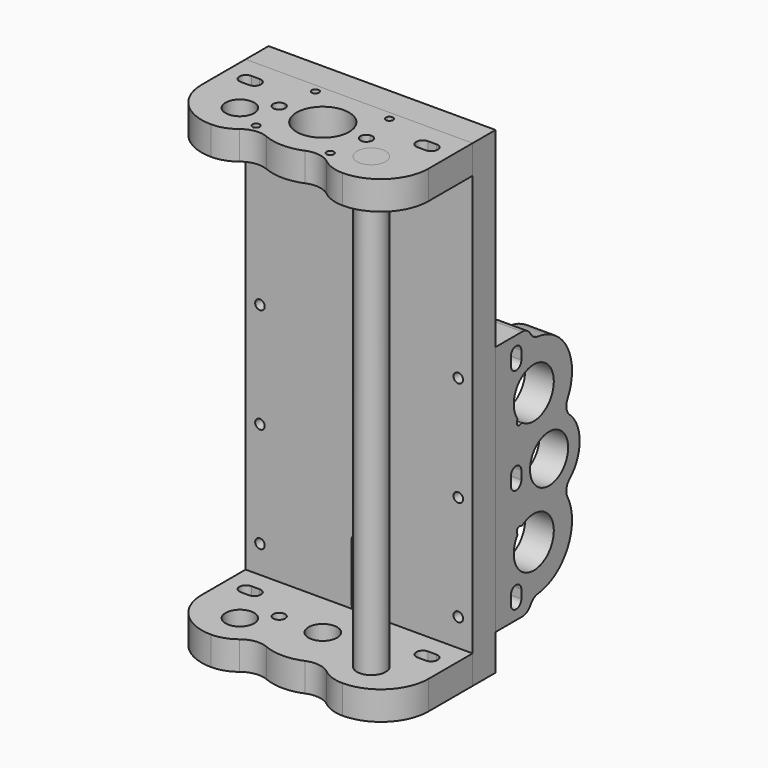
from build123d import *

# Parameters (mm, degrees)
F1_DEPTH       = 12
F2_R           = 11
F2_R_2         = 5.975
F3_DEPTH       = 12
F4_R           = 10
F5_R           = 6
F6_DEPTH       = 188
F7_R           = 9.975
F8_DEPTH       = 12
F9_R           = 2.5
F9_R_2         = 6
F9_R_3         = 5.9749995874
F10_DEPTH      = 12
F11_R          = 2
F12_DEPTH      = 25
F12_DEPTH_BACK = 10
F13_R          = 1.5
F14_DEPTH      = 25
F15_R          = 5
F16_R          = 5


# Not quite as in the source:
# - ends of sketch curves that miss each other by under 0.0002 mm in the source are joined


with BuildPart() as f1:
    # F0 (on Front) → F1 (new body)
    with BuildSketch(Plane.XZ):
        Polygon((-47.5, 1.6334e-06), (47.5, -1.6334e-06), (47.5, 200.0000016334), (-47.5, 200.0000016334), align=None)
        with BuildLine():
            ThreePointArc((3.25, 14), (0, 10.75), (-3.25, 14))
            Line((-3.25, 14), (-3.25, 37))
            ThreePointArc((-3.25, 37), (0, 40.25), (3.25, 37))
            Line((3.25, 37), (3.25, 14))
        make_face(mode=Mode.SUBTRACT)
        with BuildLine():
            ThreePointArc((-3.25, 186.0000016334), (0, 189.2500016334), (3.25, 186.0000016334))
            Line((3.25, 186.0000016334), (3.25, 163.0000016334))
            ThreePointArc((3.25, 163.0000016334), (0, 159.7500016334), (-3.25, 163.0000016334))
            Line((-3.25, 163.0000016334), (-3.25, 186.0000016334))
        make_face(mode=Mode.SUBTRACT)
    extrude(amount=-F1_DEPTH)


with BuildPart() as f3:
    # F2 (on face) → F3 (new body)
    with BuildSketch(Plane.XY.offset(200.0000016334)):
        with BuildLine():
            Line((-8.94427191, 0), (-47.5, 0))
            Line((-47.5, 0), (-47.5, -23))
            ThreePointArc((-47.5, -23), (-41.6421356237, -37.1421356237), (-27.5, -43))
            ThreePointArc((-27.5, -43), (-42.0677346215, -24.4249324484), (-20.5559152874, -14.7041477331))
            ThreePointArc((-20.5559152874, -14.7041477331), (-16.4808449816, -5.9853256402), (-8.94427191, 0))
        make_face()
        with BuildLine():
            ThreePointArc((-38.75, -13.5), (-41.5, -10.75), (-38.75, -8))
            Line((-38.75, -8), (-35.25, -8))
            ThreePointArc((-35.25, -8), (-32.5, -10.75), (-35.25, -13.5))
            Line((-35.25, -13.5), (-38.75, -13.5))
        make_face(mode=Mode.SUBTRACT)
        with BuildLine():
            Line((8.94427191, 0), (-8.94427191, 0))
            ThreePointArc((-8.94427191, 0), (-16.4808449816, -5.9853256402), (-20.5559152874, -14.7041477331))
            ThreePointArc((-20.5559152874, -14.7041477331), (-19.1407664776, -15.5451529548), (-17.8262976116, -16.5361663437))
            ThreePointArc((-17.8262976116, -16.5361663437), (-16.4581851727, -17.2566126005), (-15.7754847524, -18.6439462267))
            ThreePointArc((-15.7754847524, -18.6439462267), (-13.3425332649, -23.0435763253), (-12.5, -28))
            ThreePointArc((-12.5, -28), (-12.8897484194, -31.397138318), (-14.0387398336, -34.6177393974))
            ThreePointArc((-14.0387398336, -34.6177393974), (0, -40), (14.0387398336, -34.6177393974))
            ThreePointArc((14.0387398336, -34.6177393974), (12.587879498, -26.3786850603), (15.7754847524, -18.6439462267))
            ThreePointArc((15.7754847524, -18.6439462267), (16.4581851727, -17.2566126005), (17.8262976116, -16.5361663437))
            ThreePointArc((17.8262976116, -16.5361663437), (19.1407664776, -15.5451529548), (20.5559152874, -14.7041477331))
            ThreePointArc((20.5559152874, -14.7041477331), (16.4808449816, -5.9853256402), (8.94427191, 0))
        make_face()
        with Locations((0, -19)):
            Circle(F2_R, mode=Mode.SUBTRACT)
        with BuildLine():
            Line((47.5, 0), (8.94427191, 0))
            ThreePointArc((8.94427191, 0), (16.4808449816, -5.9853256402), (20.5559152874, -14.7041477331))
            ThreePointArc((20.5559152874, -14.7041477331), (35.2729894285, -15.1711015537), (42.5, -28))
            ThreePointArc((42.5, -28), (38.1066017178, -38.6066017178), (27.5, -43))
            ThreePointArc((27.5, -43), (41.6421356237, -37.1421356237), (47.5, -23))
            Line((47.5, -23), (47.5, 0))
        make_face()
        with BuildLine():
            Line((38.75, -13.5), (35.25, -13.5))
            ThreePointArc((35.25, -13.5), (32.5, -10.75), (35.25, -8))
            Line((35.25, -8), (38.75, -8))
            ThreePointArc((38.75, -8), (41.5, -10.75), (38.75, -13.5))
        make_face(mode=Mode.SUBTRACT)
        with BuildLine():
            ThreePointArc((-17.8262976116, -16.5361663437), (-19.1407664776, -15.5451529548), (-20.5559152874, -14.7041477331))
            ThreePointArc((-20.5559152874, -14.7041477331), (-19.9583397099, -25.5318202687), (-14.0387398336, -34.6177393974))
            ThreePointArc((-14.0387398336, -34.6177393974), (-12.8897484194, -31.397138318), (-12.5, -28))
            ThreePointArc((-12.5, -28), (-13.3425332649, -23.0435763253), (-15.7754847524, -18.6439462267))
            ThreePointArc((-15.7754847524, -18.6439462267), (-15.7563793273, -18.8215176745), (-15.75, -19))
            ThreePointArc((-15.75, -19), (-20.1617081329, -20.6110158331), (-17.8262976116, -16.5361663437))
        make_face()
        with BuildLine():
            ThreePointArc((-14.0387398336, -34.6177393974), (-19.9583397099, -25.5318202687), (-20.5559152874, -14.7041477331))
            ThreePointArc((-20.5559152874, -14.7041477331), (-42.0677346215, -24.4249324484), (-27.5, -43))
            ThreePointArc((-27.5, -43), (-19.5711315738, -40.7331475088), (-14.0387398336, -34.6177393974))
        make_face()
        with Locations((-27.5, -28)):
            Circle(F2_R_2, mode=Mode.SUBTRACT)
        with BuildLine():
            ThreePointArc((42.5, -28), (35.2729894285, -15.1711015537), (20.5559152874, -14.7041477331))
            ThreePointArc((20.5559152874, -14.7041477331), (19.9583397099, -25.5318202687), (14.0387398336, -34.6177393974))
            ThreePointArc((14.0387398336, -34.6177393974), (19.5711315738, -40.7331475088), (27.5, -43))
            ThreePointArc((27.5, -43), (38.1066017178, -38.6066017178), (42.5, -28))
        make_face()
        with Locations((27.5, -28)):
            Circle(F2_R_2, mode=Mode.SUBTRACT)
        with BuildLine():
            ThreePointArc((14.0387398336, -34.6177393974), (19.9583397099, -25.5318202687), (20.5559152874, -14.7041477331))
            ThreePointArc((20.5559152874, -14.7041477331), (19.1407664776, -15.5451529548), (17.8262976116, -16.5361663437))
            ThreePointArc((17.8262976116, -16.5361663437), (19.8610158331, -17.0882918671), (20.75, -19))
            ThreePointArc((20.75, -19), (18.0715176745, -21.4936206727), (15.7754847524, -18.6439462267))
            ThreePointArc((15.7754847524, -18.6439462267), (12.587879498, -26.3786850603), (14.0387398336, -34.6177393974))
        make_face()
    extrude(amount=-F3_DEPTH)

    # F4
    f4_edges = [f3.edges().sort_by_distance(p)[0] for p in [
        (-14.03874, -34.617739, 194.000002),
        (14.03874, -34.617739, 194.000002),
    ]]
    fillet(f4_edges, radius=F4_R)


with BuildPart() as f6:
    # F5 (on face) → F6 (new body)
    with BuildSketch(Plane.XY.offset(200.0000016334)):
        with Locations((27.5, -28)):
            Circle(F5_R)
    extrude(amount=-F6_DEPTH)


with BuildPart() as f8:
    # F7 (on face) → F8 (new body)
    with BuildSketch(Plane.YZ.offset(47.5)):
        with BuildLine():
            Line((28.5, 14.9999964573), (32, 19.9999983666))
            ThreePointArc((32, 19.9999983666), (46.1421356237, 25.8578627429), (52, 39.9999983666))
            ThreePointArc((52, 39.9999983666), (50.7273420335, 47.0204442471), (47.071333964, 53.1474274897))
            ThreePointArc((47.071333964, 53.1474274897), (56, 67.4999964573), (47.071333964, 81.8525654249))
            ThreePointArc((47.071333964, 81.8525654249), (50.7273420335, 87.9795486675), (52, 94.9999945479))
            ThreePointArc((52, 94.9999945479), (46.1421356237, 109.1421301717), (32, 114.9999945479))
            Line((32, 114.9999945479), (28.5, 119.9999964573))
            Line((28.5, 119.9999964573), (12, 119.9999964573))
            Line((12, 119.9999964573), (12, 14.9999964573))
            Line((12, 14.9999964573), (28.5, 14.9999964573))
        make_face()
        with BuildLine():
            ThreePointArc((20, 25.2499964573), (22.75, 27.9999964573), (25.5, 25.2499964573))
            Line((25.5, 25.2499964573), (25.5, 21.7499964573))
            ThreePointArc((25.5, 21.7499964573), (22.75, 18.9999964573), (20, 21.7499964573))
            Line((20, 21.7499964573), (20, 25.2499964573))
        make_face(mode=Mode.SUBTRACT)
        with BuildLine():
            ThreePointArc((26.2943182564, 48.7846907824), (39.4069435329, 32.5930548337), (23.2153075842, 45.7056801102))
            ThreePointArc((23.2153075842, 45.7056801102), (23.3755438907, 46.2028582229), (23.2632266648, 46.7130019187))
            ThreePointArc((23.2632266648, 46.7130019187), (23.5323962953, 48.4676020713), (25.286996448, 48.7367717018))
            ThreePointArc((25.286996448, 48.7367717018), (25.7971401438, 48.6244544759), (26.2943182564, 48.7846907824))
        make_face(mode=Mode.SUBTRACT)
        with BuildLine():
            Line((20, 65.5727162957), (20, 69.0727162957))
            ThreePointArc((20, 69.0727162957), (22.75, 71.8227162957), (25.5, 69.0727162957))
            Line((25.5, 69.0727162957), (25.5, 65.5727162957))
            ThreePointArc((25.5, 65.5727162957), (22.75, 62.8227162957), (20, 65.5727162957))
        make_face(mode=Mode.SUBTRACT)
        with Locations((40, 67.4999964573)):
            Circle(F7_R, mode=Mode.SUBTRACT)
        with BuildLine():
            Line((25.5, 113.2499964573), (25.5, 109.7499964573))
            ThreePointArc((25.5, 109.7499964573), (22.75, 106.9999964573), (20, 109.7499964573))
            Line((20, 109.7499964573), (20, 113.2499964573))
            ThreePointArc((20, 113.2499964573), (22.75, 115.9999964573), (25.5, 113.2499964573))
        make_face(mode=Mode.SUBTRACT)
        with BuildLine():
            ThreePointArc((23.2632266648, 88.2869909959), (23.3755438907, 88.7971346917), (23.2153075842, 89.2943128043))
            ThreePointArc((23.2153075842, 89.2943128043), (39.4069435329, 102.4069380809), (26.2943182564, 86.2153021321))
            ThreePointArc((26.2943182564, 86.2153021321), (25.7971401438, 86.3755384387), (25.286996448, 86.2632212128))
            ThreePointArc((25.286996448, 86.2632212128), (23.5323962953, 86.5323908432), (23.2632266648, 88.2869909959))
        make_face(mode=Mode.SUBTRACT)
    extrude(amount=-F8_DEPTH)


with BuildPart() as f10:
    # F9 (on face) → F10 (new body)
    with BuildSketch(Plane(origin=(0, 0, 0), x_dir=(1, 0, -3.44e-08), z_dir=(-3.44e-08, 0, -1))):
        with BuildLine():
            Line((-47.5000064647, 23), (-47.5000064647, 0))
            Line((-47.5000064647, 0), (47.4999935353, 0))
            Line((47.4999935353, 0), (47.4999935353, 23))
            ThreePointArc((47.4999935353, 23), (41.642129159, 37.1421356237), (27.4999935353, 43))
            ThreePointArc((27.4999935353, 43), (22.5678605243, 42.1659474809), (18.1842156084, 39.7565424044))
            ThreePointArc((18.1842156084, 39.7565424044), (13.3370530388, 37.6876102135), (8.1112120582, 38.3702898114))
            ThreePointArc((8.1112120582, 38.3702898114), (-6.8774e-06, 40), (-8.111225813, 38.3702898114))
            ThreePointArc((-8.111225813, 38.3702898114), (-13.3370667935, 37.6876102135), (-18.1842293632, 39.7565424044))
            ThreePointArc((-18.1842293632, 39.7565424044), (-22.5678742791, 42.1659474809), (-27.5000068774, 43))
            ThreePointArc((-27.5000068774, 43), (-41.6421420885, 37.1421356237), (-47.5000064647, 23))
        make_face()
        with BuildLine():
            Line((-35.2500064647, 8), (-38.7500064647, 8))
            ThreePointArc((-38.7500064647, 8), (-41.5000064647, 10.75), (-38.7500064647, 13.5))
            Line((-38.7500064647, 13.5), (-35.2500064647, 13.5))
            ThreePointArc((-35.2500064647, 13.5), (-32.5000064647, 10.75), (-35.2500064647, 8))
        make_face(mode=Mode.SUBTRACT)
        with Locations((-18.2500068774, 19)):
            Circle(F9_R, mode=Mode.SUBTRACT)
        with Locations((-6.8774e-06, 19)):
            Circle(F9_R_2, mode=Mode.SUBTRACT)
        with Locations((18.2499931226, 19)):
            Circle(F9_R, mode=Mode.SUBTRACT)
        with BuildLine():
            ThreePointArc((35.2499935353, 8), (32.4999935353, 10.75), (35.2499935353, 13.5))
            Line((35.2499935353, 13.5), (38.7499935353, 13.5))
            ThreePointArc((38.7499935353, 13.5), (41.4999935353, 10.75), (38.7499935353, 8))
            Line((38.7499935353, 8), (35.2499935353, 8))
        make_face(mode=Mode.SUBTRACT)
        with Locations((-27.5000068774, 28)):
            Circle(F9_R_3, mode=Mode.SUBTRACT)
        with Locations((27.4999931226, 28)):
            Circle(F9_R_3, mode=Mode.SUBTRACT)
    extrude(amount=-F10_DEPTH)


with BuildPart() as f12_tool:
    # F11 (on face) → F12 (new body, two sides)
    with BuildSketch(Plane(origin=(0, 12, 0), x_dir=(-1, 0, 0), z_dir=(0, 1, 0))) as f12_sk:
        with Locations((-37, 194.0000016334)):
            Circle(F11_R)
        with Locations((37, 194.0000016334)):
            Circle(F11_R)
        with Locations((37, 6.0000016334)):
            Circle(F11_R)
        with Locations((-37, 6.0000016334)):
            Circle(F11_R)
        with Locations((-41.5, 23.4999987879)):
            Circle(F11_R)
        with Locations((-41.5, 111.4999987879)):
            Circle(F11_R)
        with Locations((-41.5, 67.4999987879)):
            Circle(F11_R)
        with Locations((41.5, 23.4999987879)):
            Circle(F11_R)
        with Locations((41.5, 111.4999987879)):
            Circle(F11_R)
        with Locations((41.5, 67.4999987879)):
            Circle(F11_R)
    extrude(amount=-F12_DEPTH)
    extrude(f12_sk.sketch, amount=F12_DEPTH_BACK)


with BuildPart() as f1_1:
    add(f1.part)

    # F12: cut by f12_tool
    add(f12_tool.part, mode=Mode.SUBTRACT)


with BuildPart() as f3_1:
    add(f3.part)

    # F12: cut by f12_tool
    add(f12_tool.part, mode=Mode.SUBTRACT)

    # F13 (on face) → F14 (cut)
    with BuildSketch(Plane.XY.offset(200.0000016334)):
        with Locations((-15.5, -3.5)):
            Circle(F13_R)
        with Locations((-15.5, -34.5)):
            Circle(F13_R)
        with Locations((15.5, -34.5)):
            Circle(F13_R)
        with Locations((15.5, -3.5)):
            Circle(F13_R)
    extrude(amount=-F14_DEPTH, mode=Mode.SUBTRACT)


with BuildPart() as f8_1:
    add(f8.part)

    # F12: cut by f12_tool
    add(f12_tool.part, mode=Mode.SUBTRACT)

    # F15
    f15_edges = [f8_1.edges().sort_by_distance(p)[0] for p in [
        (41.5, 32, 19.999998),
        (41.5, 28.5, 14.999996),
        (41.5, 32, 114.999995),
        (41.5, 28.5, 119.999996),
    ]]
    fillet(f15_edges, radius=F15_R)

    # F16
    f16_edges = [f8_1.edges().sort_by_distance(p)[0] for p in [
        (41.5, 47.071334, 81.852565),
        (41.5, 47.071334, 53.147427),
        (41.5, 49.975, 67.499996),
    ]]
    fillet(f16_edges, radius=F16_R)


with BuildPart() as f10_1:
    add(f10.part)

    # F12: cut by f12_tool
    add(f12_tool.part, mode=Mode.SUBTRACT)


solid = Compound([f6.part, f1_1.part, f3_1.part, f8_1.part, f10_1.part])
